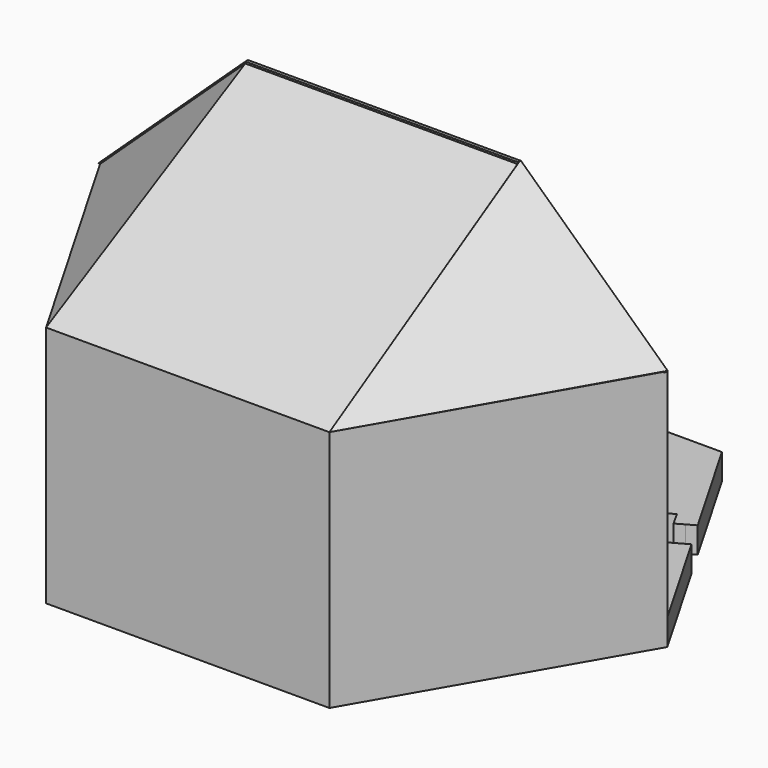
from build123d import *

# Parameters (mm, degrees)
F0_W      = 50
F0_H      = 12.5
F1_DEPTH  = 8
F2_DEPTH  = 75
F4_DEPTH  = 8
F7_DEPTH  = 3
F8_DEPTH  = 1
F11_DEPTH = 3
F14_DEPTH = 3
F15_DEPTH = 8
F16_DEPTH = 25
F17_DEPTH = 8


# Not quite as in the source:
# - a feature names something its author has since deleted; it is built from what else it names


with BuildPart() as f1:
    # F0 (on Top) → F1 (new body)
    with BuildSketch(Plane.XY):
        Polygon((-42.0179491924, 72.7772228311), (-60.5095952989, 40.7487522591), (-57.9695070384, 39.3207329262), (-55.5194165334, 43.6791064608), (-50.2642610162, 40.7248836223), (-52.7144317239, 36.366367418), (-57.615009792, 27.6494680496), (-60.0654171506, 23.2910848888), (-65.3204122546, 26.2455930623), (-62.870004896, 30.6039762231), (-65.5097997054, 32.0881441788), (-84.0358983849, 0), (-42.0179491924, -72.7772228311), (42.0179491924, -72.7772228311), (84.0358983849, 0), (65.5097997054, 32.0881441788), (62.870004896, 30.6039762231), (65.3204122546, 26.2455930623), (60.0654171506, 23.2910848888), (57.615009792, 27.6494680496), (55.164720758, 32.0079177338), (52.7144317239, 36.366367418), (50.2642610162, 40.7248836223), (55.5194165334, 43.6791064608), (57.9695070384, 39.3207329262), (60.5095952989, 40.7487522591), (42.0179491924, 72.7772228311), align=None)
        with Locations((0, 54.5829171234)):
            Rectangle(F0_W, F0_H, mode=Mode.SUBTRACT)
    extrude(amount=F1_DEPTH)

    # F0 (on Top) → F2 (join)
    with BuildSketch(Plane.XY):
        Polygon((43.75, -75.7772228311), (87.5, 0), (84.0358983849, 0), (42.0179491924, -72.7772228311), (-42.0179491924, -72.7772228311), (-84.0358983849, 0), (-87.5, 0), (-43.75, -75.7772228311), align=None)
    extrude(amount=F2_DEPTH)

    # F0 (on Top) → F4 (join)
    with BuildSketch(Plane.XY):
        Polygon((43.75, 75.7772228311), (-43.75, 75.7772228311), (-63.1248363216, 42.2190219338), (-60.5095952989, 40.7487522591), (-42.0179491924, 72.7772228311), (42.0179491924, 72.7772228311), (60.5095952989, 40.7487522591), (63.1248363216, 42.2190219338), align=None)
    extrude(amount=F4_DEPTH)

    # F6 (on face) → F7 (join)
    with BuildSketch(Plane(origin=(0, -50.1312366318, 89.3836679776), x_dir=(1, 0, 0), z_dir=(0, 0.4891706574, -0.872188092))):
        Polygon((43.75, 29.4041920927), (0, 29.4041920927), (-43.75, 29.4041920927), (-42.01795, -57.4775522498), (42.01795, -57.4775522498), align=None)
    extrude(amount=F7_DEPTH)

    # F3 (on Front) → F8 (join)
    with BuildSketch(Plane.XZ):
        Polygon((-42.01795, 114.5), (0, 114.5), (42.01795, 114.5), (84.0359, 75), (87.5, 75), (42.01795, 117.5), (0, 117.5), (-42.01795, 117.5), (-87.5, 75), (-84.0359, 75), align=None)
    extrude(amount=F8_DEPTH)

    # F10 (on face) → F11 (join)
    with BuildSketch(Plane(origin=(-67.6846727043, -39.0777640058, 72.4338274863), x_dir=(0.7723629594, -0.3015876344, 0.5590173143), z_dir=(-0.6351814378, -0.3667221741, 0.6797495039))):
        Polygon((33.2314262259, 55.789645187), (-25.6554603702, 35.6104118215), (30.9888924807, -31.0804218073), align=None)
    extrude(amount=-F11_DEPTH)

    # F13 (on face) → F14 (join)
    with BuildSketch(Plane(origin=(67.6756688636, -39.5950852503, 72.4241918832), x_dir=(0.7733047167, 0.3041472681, -0.556322078), z_dir=(-0.6340345536, 0.3709553614, -0.6785221475))):
        Polygon((-30.939509805, 30.5117392321), (-32.8751652468, -56.3649154418), (25.9400068576, -35.9776056011), align=None)
    extrude(amount=F14_DEPTH)

    # F0 (on Top) → F15 (join)
    with BuildSketch(Plane.XY):
        with Locations((0, 54.5829171234)):
            Rectangle(F0_W, F0_H)
    extrude(amount=F15_DEPTH)

    # F0 (on Top) → F16 (cut)
    with BuildSketch(Plane.XY):
        Polygon((-57.9695070384, 39.3207329262), (-60.5095952989, 40.7487522591), (-65.5097997054, 32.0881441788), (-62.870004896, 30.6039762231), (-57.615009792, 27.6494680496), (-52.7144317239, 36.366367418), align=None)
    extrude(amount=-F16_DEPTH, mode=Mode.SUBTRACT)

    # F0 (on Top) → F17 (join)
    with BuildSketch(Plane.XY):
        Polygon((-65.5097997054, 32.0881441788), (-68.125, 33.5584843966), (-87.5, 0), (-84.0358983849, 0), align=None)
        Polygon((87.5, 0), (68.125, 33.5584843966), (65.5097997054, 32.0881441788), (84.0358983849, 0), align=None)
    extrude(amount=F17_DEPTH)


solid = f1.part
